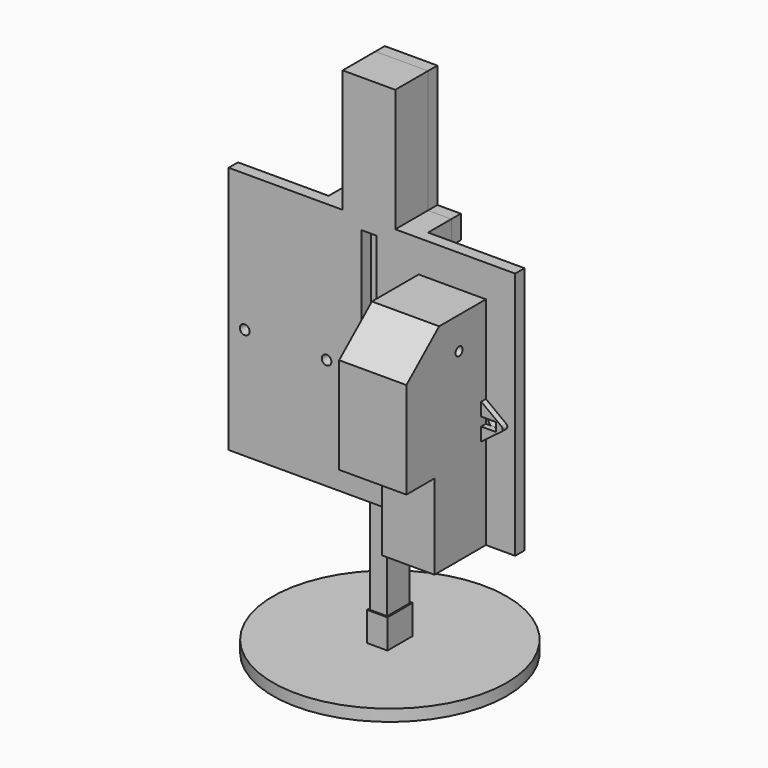
from build123d import *

# Parameters (mm, degrees)
F0_R      = 1.5
F1_DEPTH  = 23
F2_W      = 22
F2_H      = 29
F3_DEPTH  = 5
F5_DEPTH  = 2
F6_R      = 1.1
F6_R_2    = 1.65
F7_DEPTH  = 4
F8_W      = 8
F8_H      = 8
F8_R      = 1.2
F8_W_2    = 2
F8_H_2    = 4
F9_DEPTH  = 10
F10_W     = 8
F10_H     = 8
F10_R     = 1.65
F10_H_2   = 20
F10_R_2   = 1.1
F11_DEPTH = 4
F13_DEPTH = 9.6
F14_W     = 4.8
F14_H     = 15
F15_DEPTH = 25
F16_R     = 40
F17_DEPTH = 4
F18_W     = 7
F18_H     = 10.8
F18_W_2   = 6
F18_H_2   = 9.8
F19_DEPTH = 10
F20_W     = 4
F20_H     = 10
F21_DEPTH = 10


# Not quite as in the source:
# - a feature names something its author has since deleted; it is built from what else it names


with BuildPart() as f1:
    # F0 (on Right) → F1 (new body)
    with BuildSketch(Plane.YZ):
        Polygon((-22, 0), (0, 0), (0, 74), (-20, 74), (-34, 62), (-34, 29), (-22, 29), align=None)
        with Locations((-11.5, 63)):
            Circle(F0_R, mode=Mode.SUBTRACT)
    extrude(amount=F1_DEPTH)

    # F2 (on face) → F3 (cut)
    with BuildSketch(Plane(origin=(0, 0, 0), x_dir=(0, -1, 0), z_dir=(-1, 0, 0))):
        with Locations((11, 14.5)):
            Rectangle(F2_W, F2_H)
    extrude(amount=-F3_DEPTH, mode=Mode.SUBTRACT)

    # F4 (on face) → F5 (join)
    with BuildSketch(Plane(origin=(0, 0, 0), x_dir=(-1, 0, 0), z_dir=(0, 1, 0))):
        with BuildLine():
            Line((6.9333333333, 38.8), (0, 44))
            Line((0, 44), (0, 39.5))
            Line((0, 39.5), (5, 39.5))
            Line((5, 39.5), (5, 36.5))
            Line((5, 36.5), (0, 36.5))
            Line((0, 36.5), (0, 32))
            Line((0, 32), (6.9333333333, 37.2))
            ThreePointArc((6.9333333333, 37.2), (7.3333333333, 38), (6.9333333333, 38.8))
        make_face()
        with BuildLine():
            Line((-23, 39.5), (-23, 44))
            Line((-23, 44), (-29.9333333333, 38.8))
            ThreePointArc((-29.9333333333, 38.8), (-30.3333333333, 38), (-29.9333333333, 37.2))
            Line((-29.9333333333, 37.2), (-23, 32))
            Line((-23, 32), (-23, 36.5))
            Line((-23, 36.5), (-28, 36.5))
            Line((-28, 36.5), (-28, 39.5))
            Line((-28, 39.5), (-23, 39.5))
        make_face()
    extrude(amount=-F5_DEPTH)


with BuildPart() as f7:
    # F6 (on face) → F7 (new body)
    with BuildSketch(Plane(origin=(0, 0, 0), x_dir=(-1, 0, 0), z_dir=(0, 1, 0))):
        Polygon((-33, 79), (-33, 0), (65, 0), (65, 85), (26, 85), (8, 85), (-33, 85), align=None)
        with Locations((3.5, 12)):
            Circle(F6_R, mode=Mode.SUBTRACT)
        with Locations((-25.5, 38)):
            Circle(F6_R_2, mode=Mode.SUBTRACT)
        with Locations((2.5, 38)):
            Circle(F6_R_2, mode=Mode.SUBTRACT)
        with Locations((31.5, 38)):
            Circle(F6_R_2, mode=Mode.SUBTRACT)
        Polygon((14.5, 81), (17, 81), (19.5, 81), (19.5, 45), (17, 45), (14.5, 45), align=None, mode=Mode.SUBTRACT)
        with Locations((59.5, 38)):
            Circle(F6_R_2, mode=Mode.SUBTRACT)
        Polygon((8, 85), (26, 85), (26, 127), (17, 127), (8, 127), align=None)
    extrude(amount=F7_DEPTH)

    # F8 (on face) → F9 (join)
    with BuildSketch(Plane(origin=(0, 4, 0), x_dir=(-1, 0, 0), z_dir=(0, 1, 0))):
        Polygon((26, 127), (8, 127), (8, 85), (8, 77), (8, 0), (12, 0), (12, 4), (12, 123), (22, 123), (22, 4), (22, 0), (26, 0), (26, 8), (26, 77), (26, 85), align=None)
        with Locations((30, 81)):
            Rectangle(F8_W, F8_H)
        with Locations((30, 81)):
            Circle(F8_R, mode=Mode.SUBTRACT)
        with Locations((4, 81)):
            Rectangle(F8_W, F8_H)
        with Locations((4, 81)):
            Circle(F8_R, mode=Mode.SUBTRACT)
        with Locations((30, 4)):
            Rectangle(F8_W, F8_H)
        with Locations((30, 4)):
            Circle(F8_R, mode=Mode.SUBTRACT)
        with Locations((13, 2)):
            Rectangle(F8_W_2, F8_H_2)
        with Locations((21, 2)):
            Rectangle(F8_W_2, F8_H_2)
    extrude(amount=F9_DEPTH)

    # F20 (on face) → F21 (cut)
    with BuildSketch(Plane(origin=(0, 14, 0), x_dir=(-1, 0, 0), z_dir=(0, 1, 0))):
        with Locations((10, 22)):
            Rectangle(F20_W, F20_H)
    extrude(amount=-F21_DEPTH, mode=Mode.SUBTRACT)


with BuildPart() as f11:
    # F10 (on face) → F11 (new body)
    with BuildSketch(Plane(origin=(0, 14, 0), x_dir=(-1, 0, 0), z_dir=(0, 1, 0))):
        Polygon((14, 4), (14, 0), (20, 0), (20, 4), (22, 4), (22, 123), (12, 123), (12, 4), align=None)
        with Locations((30, 4)):
            Rectangle(F10_W, F10_H)
        with Locations((30, 4)):
            Circle(F10_R, mode=Mode.SUBTRACT)
        with Locations((30, 81)):
            Rectangle(F10_W, F10_H)
        with Locations((30, 81)):
            Circle(F10_R, mode=Mode.SUBTRACT)
        with Locations((4, 81)):
            Rectangle(F10_W, F10_H)
        with Locations((4, 81)):
            Circle(F10_R, mode=Mode.SUBTRACT)
        Polygon((8, 20), (8, 0), (14, 0), (14, 4), (12, 4), (12, 123), (22, 123), (22, 4), (20, 4), (20, 0), (26, 0), (26, 8), (26, 77), (26, 85), (26, 127), (8, 127), (8, 85), (8, 77), align=None)
        with Locations((4, 10)):
            Rectangle(F10_W, F10_H_2)
        with Locations((3.5, 12)):
            Circle(F10_R_2, mode=Mode.SUBTRACT)
    extrude(amount=F11_DEPTH)


with BuildPart() as f13:
    # F12 (on face) → F13 (new body)
    with BuildSketch(Plane(origin=(0, 4, 0), x_dir=(-1, 0, 0), z_dir=(0, 1, 0))):
        Polygon((19.8, 4), (17, 4), (14.2, 4), (14, -45), (19.8, -45), align=None)
        Polygon((14.2, 4), (17, 4), (19.8, 4), (21.8, 4), (21.8, 85), (12.2, 85), (12.2, 4), align=None)
    extrude(amount=F13_DEPTH)

    # F14 (on face) → F15 (cut)
    with BuildSketch(Plane.XZ.offset(-4)):
        with Locations((-17, 48.5)):
            Rectangle(F14_W, F14_H)
    extrude(amount=-F15_DEPTH, mode=Mode.SUBTRACT)


with BuildPart() as f17:
    # F16 (on face) → F17 (new body)
    with BuildSketch(Plane(origin=(0, 0, -45), x_dir=(1, 0, 0), z_dir=(0, 0, -1))):
        with Locations((-16.9, -8.8)):
            Circle(F16_R)
    extrude(amount=F17_DEPTH)

    # F18 (on face) → F19 (join)
    with BuildSketch(Plane.XY.offset(-45)):
        with Locations((-16.9, 8.8)):
            Rectangle(F18_W, F18_H)
        with Locations((-16.9, 8.8)):
            Rectangle(F18_W_2, F18_H_2, mode=Mode.SUBTRACT)
    extrude(amount=F19_DEPTH)


solid = Compound([f1.part, f7.part, f11.part, f13.part, f17.part])
